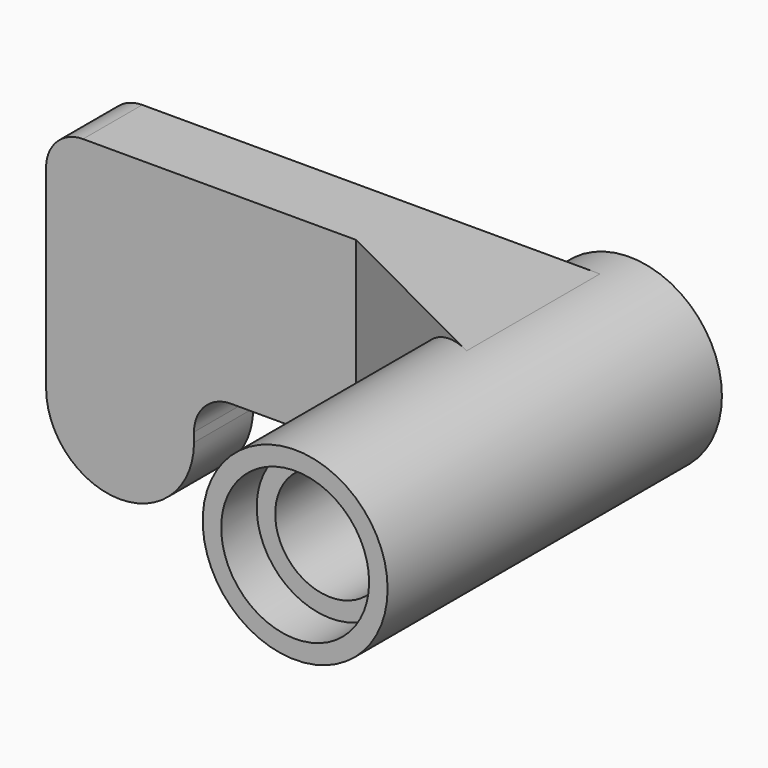
from build123d import *

# Parameters (mm, degrees)
F0_R      = 5
F1_DEPTH  = 22.6
F2_R      = 3
F3_DEPTH  = 25
F4_R      = 4
F4_R_2    = 3
F5_DEPTH  = 2.4
F7_W      = 8
F7_H      = 10
F7_H_2    = 6.5
F8_DEPTH  = 9
F10_DEPTH = 25
F11_R     = 2
F12_R     = 2
F13_R     = 3.99999


# Not quite as in the source:
# - a fillet or chamfer is up to 0.001 mm smaller than in the source, because OpenCascade refuses the exact size


with BuildPart() as f1:
    # F0 (on Front) → F1 (new body)
    with BuildSketch(Plane.XZ):
        Circle(F0_R)
    extrude(amount=F1_DEPTH)

    # F2 (on face) → F3 (cut)
    with BuildSketch(Plane.XZ.offset(22.6)):
        Circle(F2_R)
    extrude(amount=-F3_DEPTH, mode=Mode.SUBTRACT)

    # F4 (on face) → F5 (cut)
    with BuildSketch(Plane.XZ.offset(22.6)):
        Circle(F4_R)
        Circle(F4_R_2, mode=Mode.SUBTRACT)
    extrude(amount=-F5_DEPTH, mode=Mode.SUBTRACT)


with BuildPart() as f8:
    # F7 (on offset) → F8 (new body)
    with BuildSketch(Plane(origin=(0, -2, 0), x_dir=(-1, 0, 0), z_dir=(0, 1, 0))):
        with BuildLine():
            ThreePointArc((0, 5), (5, 0), (0, -5))
            Line((0, -5), (18.75, -5))
            Line((18.75, -5), (18.75, 5))
            Line((18.75, 5), (0, 5))
        make_face()
        with Locations((22.75, 0)):
            Rectangle(F7_W, F7_H)
        with Locations((22.75, -8.25)):
            Rectangle(F7_W, F7_H_2)
    extrude(amount=-F8_DEPTH)

    # F9 (on face) → F10 (cut)
    with BuildSketch(Plane.XY.offset(5)):
        Polygon((-26.75, -11), (-5, -11), (-10, -6), (-26.75, -6), align=None)
        Polygon((-10, -6), (-5, -11), (0, -11), align=None)
    extrude(amount=-F10_DEPTH, mode=Mode.SUBTRACT)

    # F11
    f11_edges = [f8.edges().sort_by_distance(p)[0] for p in [
        (-26.75, -4, 5),
    ]]
    fillet(f11_edges, radius=F11_R)

    # F12
    f12_edges = [f8.edges().sort_by_distance(p)[0] for p in [
        (-18.75, -4, -5),
    ]]
    fillet(f12_edges, radius=F12_R)

    # F13 (radius 4 in the source; OpenCascade refuses exactly that, so slightly less here)
    f13_edges = [f8.edges().sort_by_distance(p)[0] for p in [
        (-18.75, -4, -11.5),
        (-26.75, -4, -11.5),
    ]]
    fillet(f13_edges, radius=F13_R)


solid = Compound([f1.part, f8.part])
